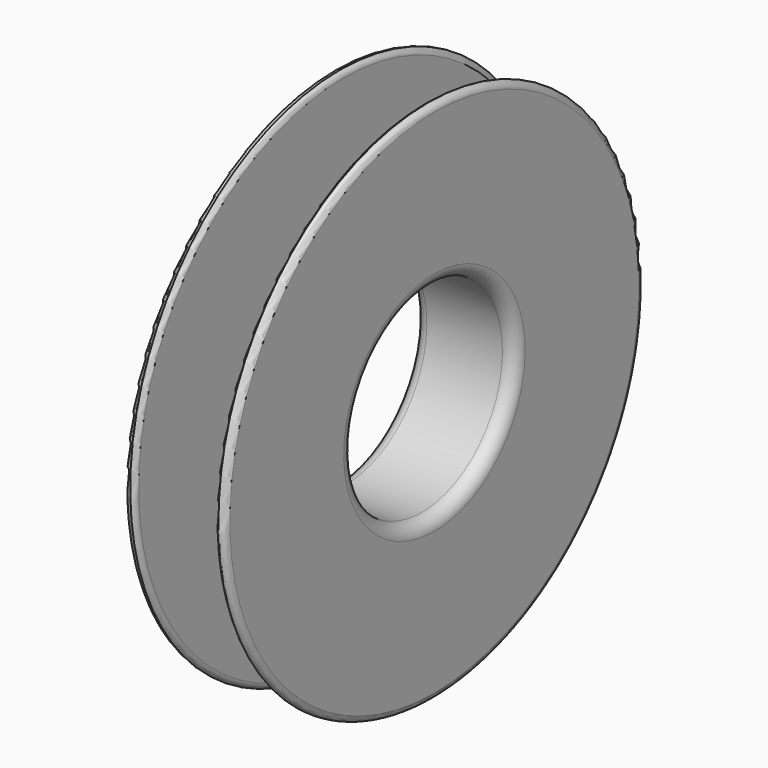
from build123d import *

# Parameters (mm, degrees)
F2_R = 2.5
F4_R = 5
F5_R = 5


# Not quite as in the source:
# - a fillet or chamfer that OpenCascade refuses, or shapes differently, is made with other operations: its cross-section is extruded or revolved along the edge and cut away or added


with BuildPart() as f1:
    # F0 (on Front) → F1 (revolve)
    with BuildSketch(Plane.XZ):
        Polygon((10, 44), (10, 40), (50, 40), (50, 44), (50, 104), (46, 104), (46, 44), (14, 44), (14, 104), (10, 104), align=None)
    revolve(axis=Axis((30, 0, 0), (1, 0, 0)))

    # F2
    f2_edges = [f1.edges().sort_by_distance(p)[0] for p in [
        (10, 0, -104),
        (50, 0, -104),
    ]]
    fillet(f2_edges, radius=F2_R)

    # F3: fillet of radius 2.5 on 2 edges, made by hand

    # F3_s1 → F3_t2 (revolve, cut)
    with BuildSketch(Plane.XZ):
        with BuildLine():
            ThreePointArc((12.5, 104), (13.5916500663, 103.0780185463), (14, 101.7087121525))
            Line((14, 101.7087121525), (14, 104))
            Line((14, 104), (12.5, 104))
        make_face()
    revolve(axis=Axis((14, 0, 0), (1, 0, 0)), mode=Mode.SUBTRACT)

    # F3_s3 → F3_t4 (revolve, cut)
    with BuildSketch(Plane.XZ):
        with BuildLine():
            ThreePointArc((47.5, 104), (46.4083499337, 103.0780185463), (46, 101.7087121525))
            Line((46, 101.7087121525), (46, 104))
            Line((46, 104), (47.5, 104))
        make_face()
    revolve(axis=Axis((46, 0, 0), (1, 0, 0)), mode=Mode.SUBTRACT)

    # F4
    f4_edges = [f1.edges().sort_by_distance(p)[0] for p in [
        (10, 0, -40),
    ]]
    fillet(f4_edges, radius=F4_R)

    # F5
    f5_edges = [f1.edges().sort_by_distance(p)[0] for p in [
        (50, 0, -40),
    ]]
    fillet(f5_edges, radius=F5_R)


solid = f1.part
